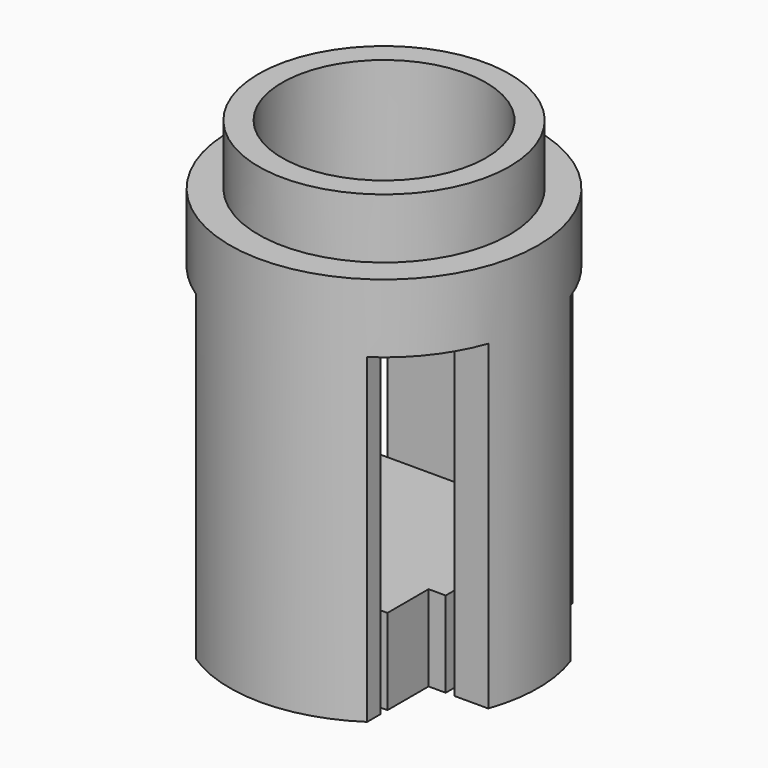
from build123d import *

# Parameters (mm, degrees)
F0_R      = 4.572
F0_R_2    = 3.0226
F1_DEPTH  = 3.81
F2_R      = 4.572
F2_R_2    = 3.7211
F3_DEPTH  = 1.778
F5_DEPTH  = 6.35
F6_DEPTH  = 3.175
F8_DEPTH  = 2.54
F11_DEPTH = 6.35
F13_DEPTH = 3.175
F14_R     = 4.8244158916
F15_DEPTH = 3.175


# Not quite as in the source:
# - after a boolean that leaves OpenCascade's solid faulty, fix() repairs it


with BuildPart() as f1:
    # F0 (on Top) → F1 (new body)
    with BuildSketch(Plane.XY):
        Circle(F0_R)
        Circle(F0_R_2, mode=Mode.SUBTRACT)
    extrude(amount=F1_DEPTH)

    # F2 (on face) → F3 (cut)
    with BuildSketch(Plane.XY.offset(3.81)):
        Circle(F2_R)
        Circle(F2_R_2, mode=Mode.SUBTRACT)
    extrude(amount=-F3_DEPTH, mode=Mode.SUBTRACT)

    # F4 (on face) → F5 (join)
    with BuildSketch(Plane(origin=(0, 0, 0), x_dir=(1, 0, 0), z_dir=(0, 0, -1))):
        with BuildLine():
            Line((-3.302, 1.524), (-4.3105229381, 1.524))
            ThreePointArc((-4.3105229381, 1.524), (-4.572, 0), (-4.3105229381, -1.524))
            Line((-4.3105229381, -1.524), (-3.302, -1.524))
            Line((-3.302, -1.524), (-3.302, 1.524))
        make_face()
        with BuildLine():
            Line((-2.54, 3.302), (2.54, 3.302))
            Line((2.54, 3.302), (2.54, 3.801523905))
            ThreePointArc((2.54, 3.801523905), (0, 4.572), (-2.54, 3.801523905))
            Line((-2.54, 3.801523905), (-2.54, 3.302))
        make_face()
        with BuildLine():
            Line((4.3105229381, 1.524), (3.302, 1.524))
            Line((3.302, 1.524), (3.302, -1.524))
            Line((3.302, -1.524), (4.3105229381, -1.524))
            ThreePointArc((4.3105229381, -1.524), (4.572, 0), (4.3105229381, 1.524))
        make_face()
        with BuildLine():
            Line((2.54, -3.801523905), (2.54, -3.302))
            Line((2.54, -3.302), (-2.54, -3.302))
            Line((-2.54, -3.302), (-2.54, -3.801523905))
            ThreePointArc((-2.54, -3.801523905), (0, -4.572), (2.54, -3.801523905))
        make_face()
    extrude(amount=F5_DEPTH)

    add(f1.part.fix(), mode=Mode.REPLACE)

    # F6 (add): faces of the model
    f6_faces = [f1.faces().sort_by_distance(p)[0] for p in [
        (0, 3.838335495, -6.35),
        (0, -3.838335495, -6.35),
        (-3.8964762164, 0, -6.35),
        (3.8964762164, 0, -6.35),
    ]]
    extrude(f6_faces, amount=F6_DEPTH)


with BuildPart() as f8:
    # F7 (on face) → F8 (new body)
    with BuildSketch(Plane(origin=(0, 0, -9.525), x_dir=(1, 0, 0), z_dir=(0, 0, -1))):
        Polygon((-2.54, 1.524), (-3.048, 1.524), (-3.048, -1.524), (-2.54, -1.524), (-2.54, -3.048), (2.54, -3.048), (2.54, -1.524), (3.048, -1.524), (3.048, 1.524), (2.54, 1.524), (2.54, 3.048), (-2.54, 3.048), align=None)
    extrude(amount=-F8_DEPTH)


with BuildPart() as f11:
    # F10 (on offset) → F11 (new body)
    with BuildSketch(Plane.XY.offset(-25.4)):
        with BuildLine():
            Line((-6.5659403285, 8.1975422484), (-4.0371337642, 3.8175207966))
            ThreePointArc((-4.0371337642, 3.8175207966), (-5.55625, 0), (-4.0371337642, -3.8175207966))
            Line((-4.0371337642, -3.8175207966), (-6.5659403285, -8.1975422484))
            Line((-6.5659403285, -8.1975422484), (-3.8163096715, -9.7850422484))
            Line((-3.8163096715, -9.7850422484), (-1.2875031072, -5.4050207966))
            ThreePointArc((-1.2875031072, -5.4050207966), (2.778125, -4.8118536498), (5.3246368714, -1.5875))
            Line((5.3246368714, -1.5875), (10.38225, -1.5875))
            Line((10.38225, -1.5875), (10.38225, 1.5875))
            Line((10.38225, 1.5875), (5.3246368714, 1.5875))
            ThreePointArc((5.3246368714, 1.5875), (2.778125, 4.8118536498), (-1.2875031072, 5.4050207966))
            Line((-1.2875031072, 5.4050207966), (-3.8163096715, 9.7850422484))
            Line((-3.8163096715, 9.7850422484), (-6.5659403285, 8.1975422484))
        make_face()
        with BuildLine():
            ThreePointArc((2.794, -3.9330080976), (0, -4.8244158916), (-2.794, -3.9330080976))
            Line((-2.794, -3.9330080976), (-2.794, -2.794))
            Line((-2.794, -2.794), (2.794, -2.794))
            Line((2.794, -2.794), (2.794, -3.9330080976))
        make_face(mode=Mode.SUBTRACT)
        with BuildLine():
            Line((-4.4850030606, 1.7775646942), (-2.7929016728, 1.7775646942))
            Line((-2.7929016728, 1.7775646942), (-2.7929016728, -1.7775646942))
            Line((-2.7929016728, -1.7775646942), (-4.4850030606, -1.7775646942))
            ThreePointArc((-4.4850030606, -1.7775646942), (-4.8244158916, 0), (-4.4850030606, 1.7775646942))
        make_face(mode=Mode.SUBTRACT)
        with BuildLine():
            Line((2.794, 2.794), (-2.794, 2.794))
            Line((-2.794, 2.794), (-2.794, 3.9330080976))
            ThreePointArc((-2.794, 3.9330080976), (0, 4.8244158916), (2.794, 3.9330080976))
            Line((2.794, 3.9330080976), (2.794, 2.794))
        make_face(mode=Mode.SUBTRACT)
        with BuildLine():
            Line((4.4850030606, -1.7775646942), (2.7929016728, -1.7775646942))
            Line((2.7929016728, -1.7775646942), (2.7929016728, 1.7775646942))
            Line((2.7929016728, 1.7775646942), (4.4850030606, 1.7775646942))
            ThreePointArc((4.4850030606, 1.7775646942), (4.8244158916, 0), (4.4850030606, -1.7775646942))
        make_face(mode=Mode.SUBTRACT)
    extrude(amount=F11_DEPTH)

    # F12 (on face) → F13 (join)
    with BuildSketch(Plane.XY.offset(-19.05)):
        with BuildLine():
            Line((10.38225, -1.5875), (10.38225, 1.5875))
            Line((10.38225, 1.5875), (5.3246368714, 1.5875))
            ThreePointArc((5.3246368714, 1.5875), (2.778125, 4.8118536498), (-1.2875031072, 5.4050207966))
            Line((-1.2875031072, 5.4050207966), (-3.8163096715, 9.7850422484))
            Line((-3.8163096715, 9.7850422484), (-6.5659403285, 8.1975422484))
            Line((-6.5659403285, 8.1975422484), (-4.0371337642, 3.8175207966))
            ThreePointArc((-4.0371337642, 3.8175207966), (-5.55625, 0), (-4.0371337642, -3.8175207966))
            Line((-4.0371337642, -3.8175207966), (-6.5659403285, -8.1975422484))
            Line((-6.5659403285, -8.1975422484), (-3.8163096715, -9.7850422484))
            Line((-3.8163096715, -9.7850422484), (-1.2875031072, -5.4050207966))
            ThreePointArc((-1.2875031072, -5.4050207966), (2.778125, -4.8118536498), (5.3246368714, -1.5875))
            Line((5.3246368714, -1.5875), (10.38225, -1.5875))
        make_face()
        with BuildLine():
            ThreePointArc((3.9330080976, -2.794), (0, -4.8244158916), (-3.9330080976, -2.794))
            Line((-3.9330080976, -2.794), (3.9330080976, -2.794))
        make_face(mode=Mode.SUBTRACT)
        with BuildLine():
            Line((4.4850030606, -1.7775646942), (-4.4850030606, -1.7775646942))
            ThreePointArc((-4.4850030606, -1.7775646942), (-4.8244158916, 0), (-4.4850030606, 1.7775646942))
            Line((-4.4850030606, 1.7775646942), (4.4850030606, 1.7775646942))
            ThreePointArc((4.4850030606, 1.7775646942), (4.8244158916, 0), (4.4850030606, -1.7775646942))
        make_face(mode=Mode.SUBTRACT)
        with BuildLine():
            Line((3.9330080976, 2.794), (-3.9330080976, 2.794))
            ThreePointArc((-3.9330080976, 2.794), (0, 4.8244158916), (3.9330080976, 2.794))
        make_face(mode=Mode.SUBTRACT)
    extrude(amount=F13_DEPTH)

    # F14 (on face) → F15 (join)
    with BuildSketch(Plane.XY.offset(-15.875)):
        with BuildLine():
            Line((10.38225, -1.5875), (10.38225, 1.5875))
            Line((10.38225, 1.5875), (5.3246368714, 1.5875))
            ThreePointArc((5.3246368714, 1.5875), (2.778125, 4.8118536498), (-1.2875031072, 5.4050207966))
            Line((-1.2875031072, 5.4050207966), (-3.8163096715, 9.7850422484))
            Line((-3.8163096715, 9.7850422484), (-6.5659403285, 8.1975422484))
            Line((-6.5659403285, 8.1975422484), (-4.0371337642, 3.8175207966))
            ThreePointArc((-4.0371337642, 3.8175207966), (-5.55625, 0), (-4.0371337642, -3.8175207966))
            Line((-4.0371337642, -3.8175207966), (-6.5659403285, -8.1975422484))
            Line((-6.5659403285, -8.1975422484), (-3.8163096715, -9.7850422484))
            Line((-3.8163096715, -9.7850422484), (-1.2875031072, -5.4050207966))
            ThreePointArc((-1.2875031072, -5.4050207966), (2.778125, -4.8118536498), (5.3246368714, -1.5875))
            Line((5.3246368714, -1.5875), (10.38225, -1.5875))
        make_face()
        Circle(F14_R, mode=Mode.SUBTRACT)
    extrude(amount=F15_DEPTH)


solid = Compound([f1.part, f8.part])
